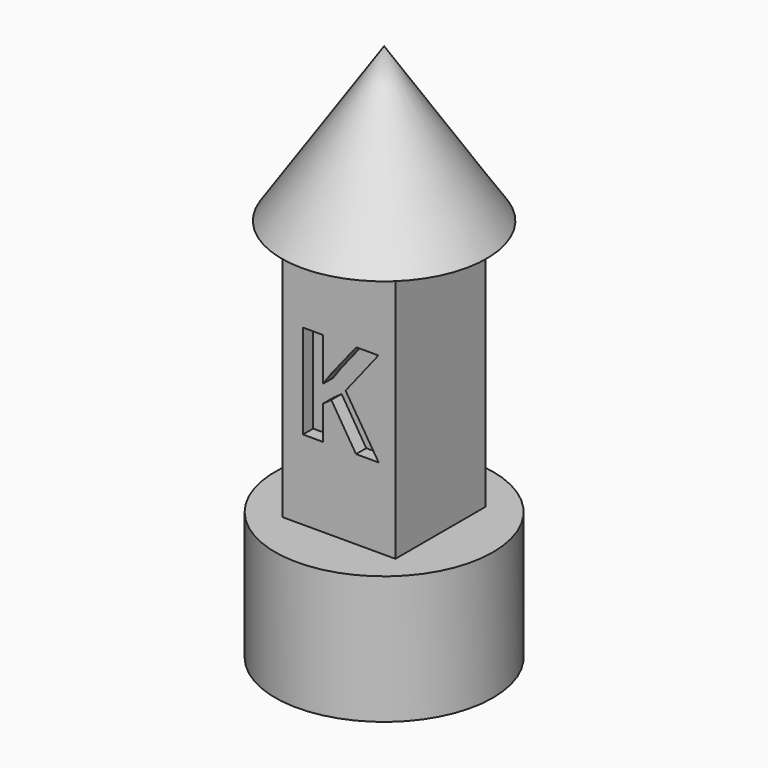
from build123d import *

# Parameters (mm, degrees)
F0_R         = 10.795
F1_DEPTH     = 12.7
F2_W         = 11.176
F2_H         = 11.176
F3_DEPTH     = 38.1
F6_TEXT_SIZE = 13.0675241158
F7_DEPTH     = 1.27


# Not quite as in the source:
# - Text() gives the source's letters only with a copy of the font that has no kerning and outlines rounded to 1/6400 em; it was checked with that copy


with BuildPart() as f1:
    # F0 (on Top) → F1 (new body)
    with BuildSketch(Plane.XY):
        Circle(F0_R)
    extrude(amount=F1_DEPTH)

    # F2 (on Top) → F3 (join)
    with BuildSketch(Plane.XY):
        Rectangle(F2_W, F2_H)
    extrude(amount=F3_DEPTH)

    # F4 (on Right) → F5 (revolve)
    with BuildSketch(Plane.YZ):
        Polygon((-10.16, 38.1), (0, 38.1), (0, 53.34), align=None)
    revolve(axis=Axis((0, 0, 45.72), (0, 0, 1)))

    # F6 (on face) → F7 (cut)
    with BuildSketch(Plane.XZ.offset(5.588)):
        with Locations((-4.7473585195, 20.5667612921)):
            Text('K', F6_TEXT_SIZE, font='Open Sans', font_style=FontStyle.BOLD, text_align=(TextAlign.LEFT, TextAlign.BOTTOM))
    extrude(amount=-F7_DEPTH, mode=Mode.SUBTRACT)


solid = f1.part
